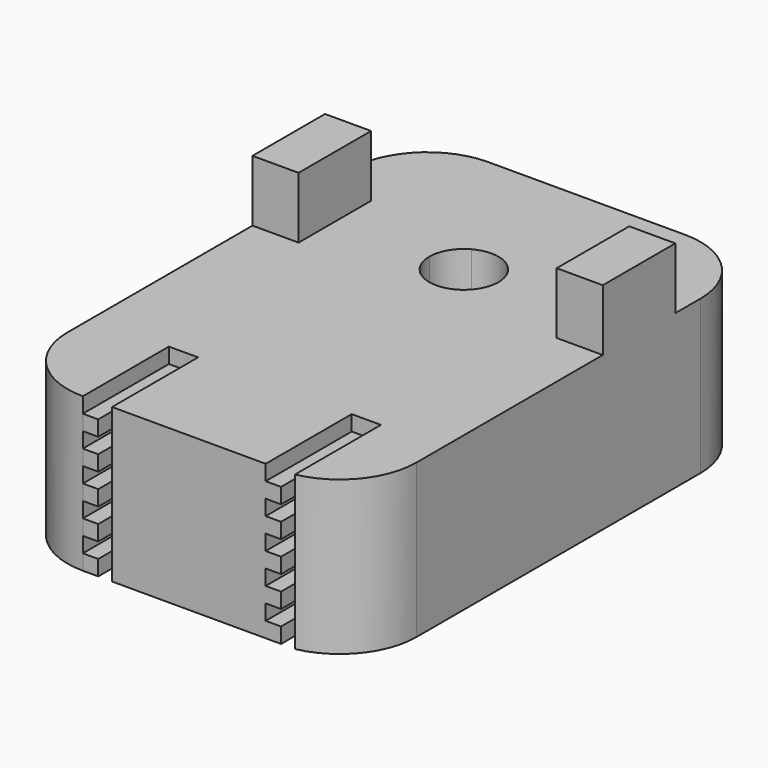
from build123d import *

# Parameters (mm, degrees)
F0_W        = 18.5
F0_H        = 13
F0_W_2      = 4.3
F0_W_3      = 3
F0_H_2      = 2.95
F1_DEPTH    = 10
F3_DEPTH    = 7
F4_T1_DEPTH = 35
F4_T3_DEPTH = 34.4948974279
F0_H_3      = 5.9
F5_DEPTH    = 14
F6_R        = 5.5
F7_DEPTH    = 4
F8_SIZE     = 2


# Not quite as in the source:
# - a fillet or chamfer that OpenCascade refuses, or shapes differently, is made with other operations: its cross-section is extruded or revolved along the edge and cut away or added


with BuildPart() as f1:
    # F0 (on Top) → F1 (new body)
    with BuildSketch(Plane.XY):
        with Locations((5.190736489, 6.5)):
            Rectangle(F0_W, F0_H)
        with Locations((16.590736489, 6.5)):
            Rectangle(F0_W_2, F0_H)
        Polygon((14.440736489, 20.05), (14.440736489, 13), (18.740736489, 13), (18.740736489, 20.05), (15.740736489, 20.05), (15.740736489, 25.95), (18.740736489, 25.95), (18.740736489, 33), (14.440736489, 33), (14.440736489, 25.95), (14.440736489, 23), align=None)
        with BuildLine():
            Line((-4.059263511, 20.05), (-4.059263511, 13))
            Line((-4.059263511, 13), (14.440736489, 13))
            Line((14.440736489, 13), (14.440736489, 20.05))
            Line((14.440736489, 20.05), (11.440736489, 20.05))
            Line((11.440736489, 20.05), (11.440736489, 23))
            Line((11.440736489, 23), (9.590736489, 23))
            ThreePointArc((9.590736489, 23), (8.4904647177, 21.0659304563), (6.265736489, 21.0234183548))
            ThreePointArc((6.265736489, 21.0234183548), (4.0410082602, 21.0659304563), (2.940736489, 23))
            Line((2.940736489, 23), (-1.059263511, 23))
            Line((-1.059263511, 23), (-1.059263511, 20.05))
            Line((-1.059263511, 20.05), (-4.059263511, 20.05))
        make_face()
        with Locations((12.940736489, 21.525)):
            Rectangle(F0_W_3, F0_H_2)
        with Locations((12.940736489, 24.475)):
            Rectangle(F0_W_3, F0_H_2)
        with BuildLine():
            Line((-4.059263511, 33), (-4.059263511, 25.95))
            Line((-4.059263511, 25.95), (-1.059263511, 25.95))
            Line((-1.059263511, 25.95), (-1.059263511, 23))
            Line((-1.059263511, 23), (2.940736489, 23))
            ThreePointArc((2.940736489, 23), (4.0410082602, 24.9340695437), (6.265736489, 24.9765816452))
            ThreePointArc((6.265736489, 24.9765816452), (8.4904647177, 24.9340695437), (9.590736489, 23))
            Line((9.590736489, 23), (11.440736489, 23))
            Line((11.440736489, 23), (11.440736489, 25.95))
            Line((11.440736489, 25.95), (14.440736489, 25.95))
            Line((14.440736489, 25.95), (14.440736489, 33))
            Line((14.440736489, 33), (-4.059263511, 33))
        make_face()
        with BuildLine():
            Line((5.090736489, 23), (2.940736489, 23))
            ThreePointArc((2.940736489, 23), (4.0410082602, 21.0659304563), (6.265736489, 21.0234183548))
            ThreePointArc((6.265736489, 21.0234183548), (5.4066669452, 21.8502717712), (5.090736489, 23))
        make_face()
        with BuildLine():
            ThreePointArc((6.265736489, 24.9765816452), (4.0410082602, 24.9340695437), (2.940736489, 23))
            Line((2.940736489, 23), (5.090736489, 23))
            ThreePointArc((5.090736489, 23), (5.4066669452, 24.1497282288), (6.265736489, 24.9765816452))
        make_face()
    extrude(amount=F1_DEPTH)

    # F2 (on face) → F3 (cut)
    with BuildSketch(Plane.XZ):
        Polygon((2.840736489, 10), (0.940736489, 10), (0.940736489, 9), (1.940736489, 9), (1.940736489, 8), (0.940736489, 8), (0.940736489, 7), (1.940736489, 7), (1.940736489, 6), (0.940736489, 6), (0.940736489, 5), (1.940736489, 5), (1.940736489, 4), (0.940736489, 4), (0.940736489, 3), (1.940736489, 3), (1.940736489, 2), (0.940736489, 2), (0.940736489, 1), (1.940736489, 1), (1.940736489, 0), (2.840736489, 0), align=None)
        Polygon((14.740736489, 10), (12.840736489, 10), (12.840736489, 9), (13.840736489, 9), (13.840736489, 8), (12.840736489, 8), (12.840736489, 7), (13.840736489, 7), (13.840736489, 6), (12.840736489, 6), (12.840736489, 5), (13.840736489, 5), (13.840736489, 4), (12.840736489, 4), (12.840736489, 3), (13.840736489, 3), (13.840736489, 2), (12.840736489, 2), (12.840736489, 1), (13.840736489, 1), (13.840736489, 0), (14.740736489, 0), align=None)
    extrude(amount=-F3_DEPTH, mode=Mode.SUBTRACT)

    # F4: fillet of radius 5 on 4 edges, made by hand

    # F4_s2 → F4_t1 (cut)
    with BuildSketch(Plane.XY.offset(-12.5)):
        with BuildLine():
            ThreePointArc((-4.059263511, 28), (-2.594797417, 31.5355339059), (0.940736489, 33))
            Line((0.940736489, 33), (-4.059263511, 33))
            Line((-4.059263511, 33), (-4.059263511, 28))
        make_face()
        with BuildLine():
            ThreePointArc((0.940736489, 0), (-2.594797417, 1.4644660941), (-4.059263511, 5))
            Line((-4.059263511, 5), (-4.059263511, 0))
            Line((-4.059263511, 0), (0.940736489, 0))
        make_face()
        with BuildLine():
            ThreePointArc((13.740736489, 33), (17.2762703949, 31.5355339059), (18.740736489, 28))
            Line((18.740736489, 28), (18.740736489, 33))
            Line((18.740736489, 33), (13.740736489, 33))
        make_face()
    extrude(amount=F4_T1_DEPTH, mode=Mode.SUBTRACT)

    # F4_s4 → F4_t3 (cut)
    with BuildSketch(Plane.XY.offset(-12.2474487139)):
        with BuildLine():
            ThreePointArc((18.740736489, 4.8989794856), (17.6137198352, 1.7367018254), (14.740736489, 0))
            Line((14.740736489, 0), (18.740736489, 0))
            Line((18.740736489, 0), (18.740736489, 4.8989794856))
        make_face()
    extrude(amount=F4_T3_DEPTH, mode=Mode.SUBTRACT)

    # F0 (on Top) → F5 (join)
    with BuildSketch(Plane.XY):
        with Locations((-2.559263511, 24.475)):
            Rectangle(F0_W_3, F0_H_2)
        with Locations((-2.559263511, 21.525)):
            Rectangle(F0_W_3, F0_H_2)
        with Locations((17.240736489, 23)):
            Rectangle(F0_W_3, F0_H_3)
    extrude(amount=F5_DEPTH)

    # F6 (on face) → F7 (cut)
    with BuildSketch(Plane(origin=(0, 0, 0), x_dir=(1, 0, 0), z_dir=(0, 0, -1))):
        with Locations((7.340736489, -23)):
            Circle(F6_R)
    extrude(amount=-F7_DEPTH, mode=Mode.SUBTRACT)

    # F8
    f8_edges = [f1.edges().sort_by_distance(p)[0] for p in [
        (1.840736, 23, 4),
    ]]
    chamfer(f8_edges, length=F8_SIZE)


solid = f1.part
